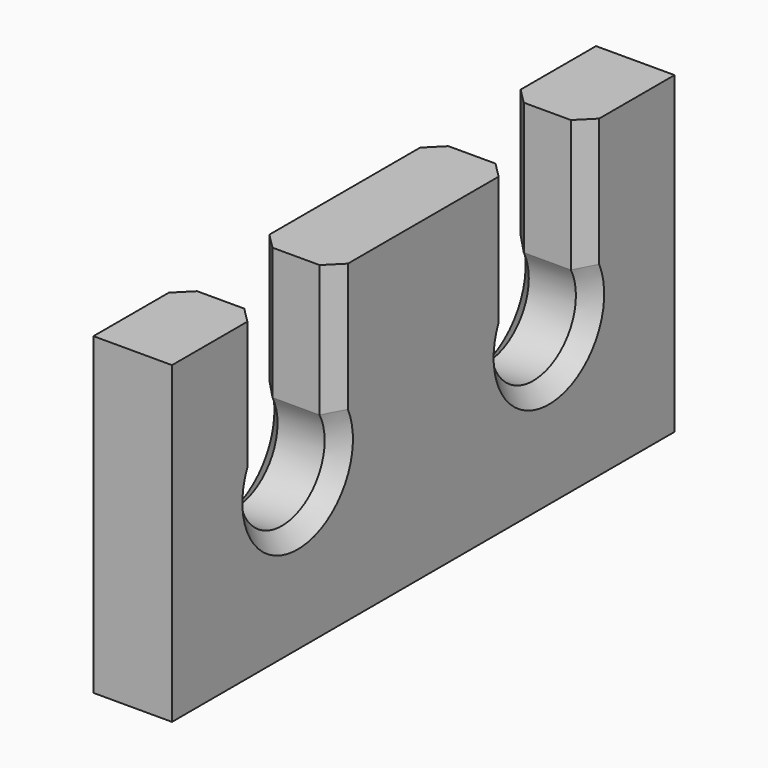
from build123d import *

# Parameters (mm, degrees)
F1_DEPTH = 6.35
F2_SIZE  = 1.27


# Not quite as in the source:
# - a feature names something its author has since deleted; it is built from what else it names


with BuildPart() as f1:
    # F0 (on Right) → F1 (new body)
    with BuildSketch(Plane.YZ):
        with BuildLine():
            Line((-10.0986241174, -8.2946426358), (40.7013758826, -8.2946426358))
            Line((40.7013758826, -8.2946426358), (40.7013758826, 17.1053573642))
            Line((40.7013758826, 17.1053573642), (31.8113758826, 17.1053573642))
            Line((31.8113758826, 17.1053573642), (31.8113758826, 6.4373573642))
            ThreePointArc((31.8113758826, 6.4373573642), (28.0013758826, 0.0873573642), (24.1913758826, 6.4373573642))
            Line((24.1913758826, 6.4373573642), (24.1913758826, 17.1053573642))
            Line((24.1913758826, 17.1053573642), (15.3013758826, 17.1053573642))
            Line((15.3013758826, 17.1053573642), (6.4113758826, 17.1053573642))
            Line((6.4113758826, 17.1053573642), (6.4113758826, 6.4373573642))
            ThreePointArc((6.4113758826, 6.4373573642), (2.6013758826, 0.0873573642), (-1.2086241174, 6.4373573642))
            Line((-1.2086241174, 6.4373573642), (-1.2086241174, 17.1053573642))
            Line((-1.2086241174, 17.1053573642), (-10.0986241174, 17.1053573642))
            Line((-10.0986241174, 17.1053573642), (-10.0986241174, -8.2946426358))
        make_face()
    extrude(amount=F1_DEPTH)

    # F2
    f2_edges = [f1.edges().sort_by_distance(p)[0] for p in [
        (6.35, -1.208624, 11.771357),
        (6.35, 2.601376, 0.087357),
        (6.35, 6.411376, 11.771357),
        (6.35, 24.191376, 11.771357),
        (6.35, 28.001376, 0.087357),
        (6.35, 31.811376, 11.771357),
        (0, 2.601376, 0.087357),
        (0, -1.208624, 11.771357),
        (0, 24.191376, 11.771357),
        (0, 28.001376, 0.087357),
        (0, 31.811376, 11.771357),
        (0, 6.411376, 11.771357),
    ]]
    chamfer(f2_edges, length=F2_SIZE)


solid = f1.part
